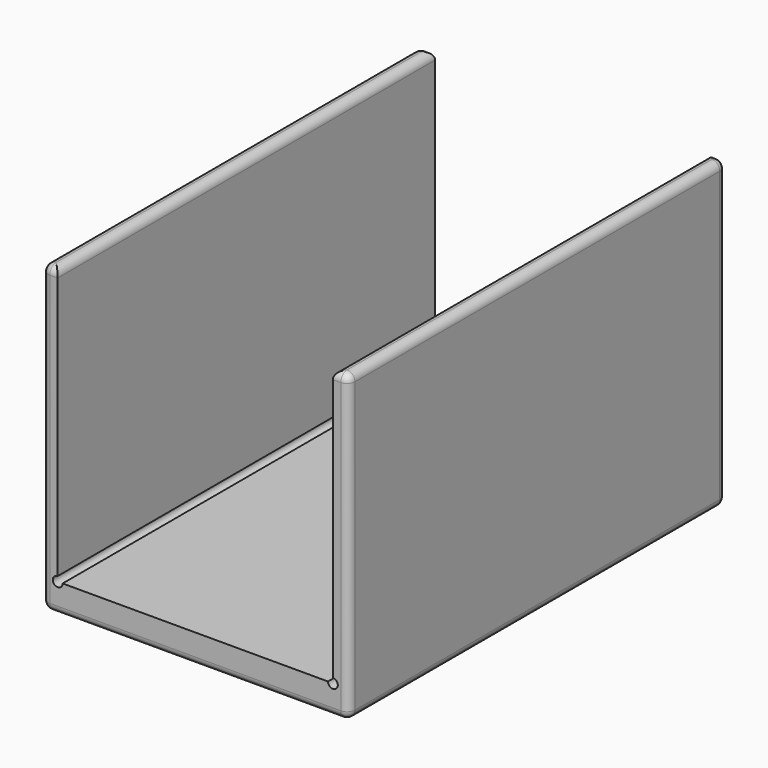
from build123d import *

# Parameters (mm, degrees)
F1_DEPTH = 76.2
F2_R     = 1.26999


# Not quite as in the source:
# - a fillet or chamfer is up to 0.001 mm smaller than in the source, because OpenCascade refuses the exact size


with BuildPart() as f1:
    # F0 (on Front) → F1 (new body)
    with BuildSketch(Plane.XZ):
        with BuildLine():
            Line((-22.225, 19.05), (-24.765, 19.05))
            Line((-24.765, 19.05), (-24.765, -30.1625))
            Line((-24.765, -30.1625), (0, -30.1625))
            Line((0, -30.1625), (0, -25.4))
            Line((0, -25.4), (-21.43125, -25.4))
            ThreePointArc((-21.43125, -25.4), (-22.7862660076, -25.9612660076), (-22.225, -24.60625))
            Line((-22.225, -24.60625), (-22.225, 19.05))
        make_face()
        with BuildLine():
            Line((0, -25.4), (0, -30.1625))
            Line((0, -30.1625), (24.765, -30.1625))
            Line((24.765, -30.1625), (24.765, 19.05))
            Line((24.765, 19.05), (22.225, 19.05))
            Line((22.225, 19.05), (22.225, -24.60625))
            ThreePointArc((22.225, -24.60625), (22.7862660076, -24.8387339924), (23.01875, -25.4))
            ThreePointArc((23.01875, -25.4), (22.225, -26.19375), (21.43125, -25.4))
            Line((21.43125, -25.4), (0, -25.4))
        make_face()
    extrude(amount=F1_DEPTH)

    # F2 (radius 1.27 in the source; OpenCascade refuses exactly that, so slightly less here)
    f2_edges = [f1.edges().sort_by_distance(p)[0] for p in [
        (24.765, -38.1, 19.05),
        (22.225, -38.1, 19.05),
        (23.495, 0, 19.05),
        (23.495, -76.2, 19.05),
        (-22.225, -38.1, 19.05),
        (-24.765, -38.1, 19.05),
        (-23.495, 0, 19.05),
        (-23.495, -76.2, 19.05),
        (-24.765, -76.2, -5.55625),
        (24.765, -76.2, -5.55625),
        (24.765, 0, -5.55625),
        (-24.765, 0, -5.55625),
        (-24.765, -38.1, -30.1625),
        (24.765, -38.1, -30.1625),
        (0, 0, -30.1625),
        (0, -76.2, -30.1625),
    ]]
    fillet(f2_edges, radius=F2_R)


solid = f1.part
